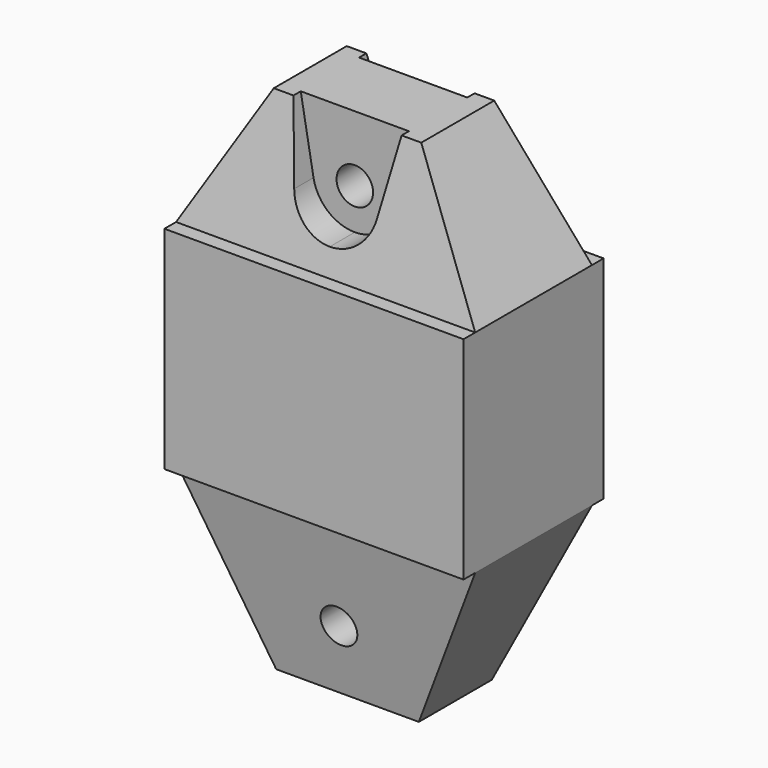
from build123d import *

# Parameters (mm, degrees)
F1_DEPTH = 82
F2_R     = 5
F3_DEPTH = 48
F5_DEPTH = 14


# Not quite as in the source:
# - a pattern or mirror of a feature is missing from the dataset's text; its kind, count and spacing are read off the source's solid


with BuildPart() as f1:
    # F0 (on Right) → F1 (new body)
    with BuildSketch(Plane.YZ):
        Polygon((12.5, 65), (-12.5, 65), (-20, 29), (-24, 29), (-24, -29), (-20, -29), (-12.5, -75), (12.5, -75), (20, -29), (24, -29), (24, 29), (20, 29), align=None)
    extrude(amount=F1_DEPTH)

    # F2 (on face) → F3 (intersect, through all)
    with BuildSketch(Plane(origin=(0, 24, 0), x_dir=(-1, 0, 0), z_dir=(0, 1, 0))):
        Polygon((-26.5581123827, 75), (-55.4418876173, 75), (-92, 11.6794919243), (-92, -7.5549307949), (-55.8867711433, -85), (-26.1132288567, -85), (10, -7.5549307949), (10, 11.6794919243), align=None)
        with Locations((-41, -57)):
            Circle(F2_R, mode=Mode.SUBTRACT)
        with Locations((-41, 47)):
            Circle(F2_R, mode=Mode.SUBTRACT)
    extrude(amount=-F3_DEPTH, mode=Mode.INTERSECT)

    # F4 (on face) → F5 (cut)
    with BuildSketch(Plane(origin=(0, 24, 0), x_dir=(-1, 0, 0), z_dir=(0, 1, 0))):
        with BuildLine():
            ThreePointArc((-52.3229859469, 45.2858959478), (-48.3869925151, 38.4821097444), (-41, 35.7958683968))
            Line((-41, 35.7958683968), (-41, 66))
            Line((-41, 66), (-56, 66))
            Line((-56, 66), (-52.3229859469, 45.2858959478))
        make_face()
        with BuildLine():
            Line((-41, 66), (-41, 35.7958683968))
            ThreePointArc((-41, 35.7958683968), (-33.6130074849, 38.4821097444), (-29.6770140531, 45.2858959478))
            Line((-29.6770140531, 45.2858959478), (-26, 66))
            Line((-26, 66), (-41, 66))
        make_face()
    f5 = extrude(amount=-F5_DEPTH, mode=Mode.SUBTRACT)

    # F5_copies: F5 across plane
    add(f5.mirror(Plane(origin=(0, 0, 0), x_dir=(0, 0, -1), z_dir=(0, -1, 0))), mode=Mode.SUBTRACT)


solid = f1.part
